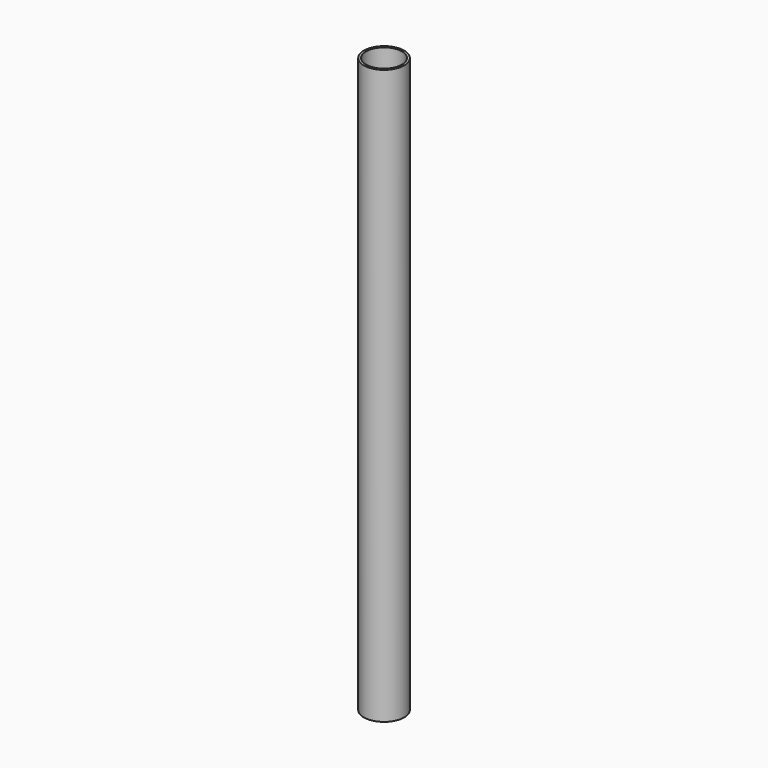
from build123d import *

# Parameters (mm, degrees)
F0_R     = 14.2875
F0_R_2   = 12.7
F1_DEPTH = 406.4


# Not quite as in the source:
# - a feature names something its author has since deleted; it is built from what else it names


with BuildPart() as f1:
    # F0 (on Top) → F1 (new body)
    with BuildSketch(Plane.XY):
        Circle(F0_R)
        Circle(F0_R_2, mode=Mode.SUBTRACT)
    extrude(amount=F1_DEPTH)


solid = f1.part
